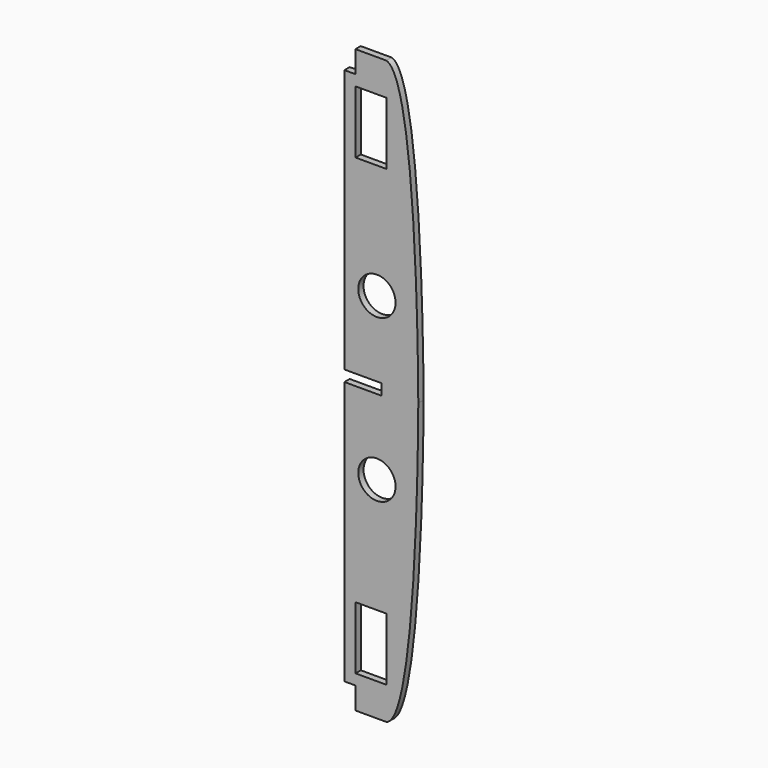
from build123d import *

# Parameters (mm, degrees)
F0_R     = 16.9272487263
F0_W     = 28.0263870955
F0_H     = 56.8133033812
F1_DEPTH = 6


# Not quite as in the source:
# - a feature names something its author has since deleted; it is built from what else it names


with BuildPart() as f1:
    # F0 (on Front) → F1 (new body)
    with BuildSketch(Plane.XZ):
        with BuildLine():
            add(Edge.make_bspline(
                [(181.3542903333, 259), (206.5942975175, 252.0158164026), (209.7991991798, 56.7803677557), (210.2653369369, 6.6428164877)],
                knots=[0, 0, 0, 0, 231.86444259, 231.86444259, 231.86444259, 231.86444259], degree=3))
            Line((181.3542903333, 259), (153.3542903333, 259))
            Line((153.3542903333, 259), (153.3542903333, 239))
            Line((153.3542903333, 239), (143.3542903333, 239))
            Line((143.3542903333, 239), (143.3542903333, 0))
            Line((143.3542903333, 0), (176.8542903333, 0))
            Line((176.8542903333, 0), (176.8542903333, -5))
            Line((176.8542903333, -5), (210.3542903333, -5))
            add(Edge.make_bspline(
                [(210.2653369369, 6.6428164877), (210.3331344644, -0.6494527163), (210.3429952934, -4.8722740171), (210.3542903333, -5)],
                knots=[231.86444259, 231.86444259, 231.86444259, 231.86444259, 265.5880268386, 265.5880268386, 265.5880268386, 265.5880268386], degree=3))
        make_face()
        with Locations((172.8220252337, 68.3807536824)):
            Circle(F0_R, mode=Mode.SUBTRACT)
        with Locations((167.491195113, 200.8973438895)):
            Rectangle(F0_W, F0_H, mode=Mode.SUBTRACT)
        with BuildLine():
            add(Edge.make_bspline(
                [(210.2653369369, -16.6428164877), (210.3331344644, -9.3505472837), (210.3429952934, -5.1277259829), (210.3542903333, -5)],
                knots=[231.86444259, 231.86444259, 231.86444259, 231.86444259, 265.5880268386, 265.5880268386, 265.5880268386, 265.5880268386], degree=3))
            Line((210.3542903333, -5), (176.8542903333, -5))
            Line((176.8542903333, -5), (176.8542903333, -10))
            Line((176.8542903333, -10), (143.3542903333, -10))
            Line((143.3542903333, -10), (143.3542903333, -249))
            Line((143.3542903333, -249), (153.3542903333, -249))
            Line((153.3542903333, -249), (153.3542903333, -269))
            Line((153.3542903333, -269), (181.3542903333, -269))
            add(Edge.make_bspline(
                [(181.3542903333, -269), (206.5942975175, -262.0158164026), (209.7991991798, -66.7803677557), (210.2653369369, -16.6428164877)],
                knots=[0, 0, 0, 0, 231.86444259, 231.86444259, 231.86444259, 231.86444259], degree=3))
        make_face()
        with Locations((167.491195113, -210.8973438895)):
            Rectangle(F0_W, F0_H, mode=Mode.SUBTRACT)
        with Locations((172.8220252337, -78.3807536824)):
            Circle(F0_R, mode=Mode.SUBTRACT)
    extrude(amount=F1_DEPTH)


solid = f1.part
